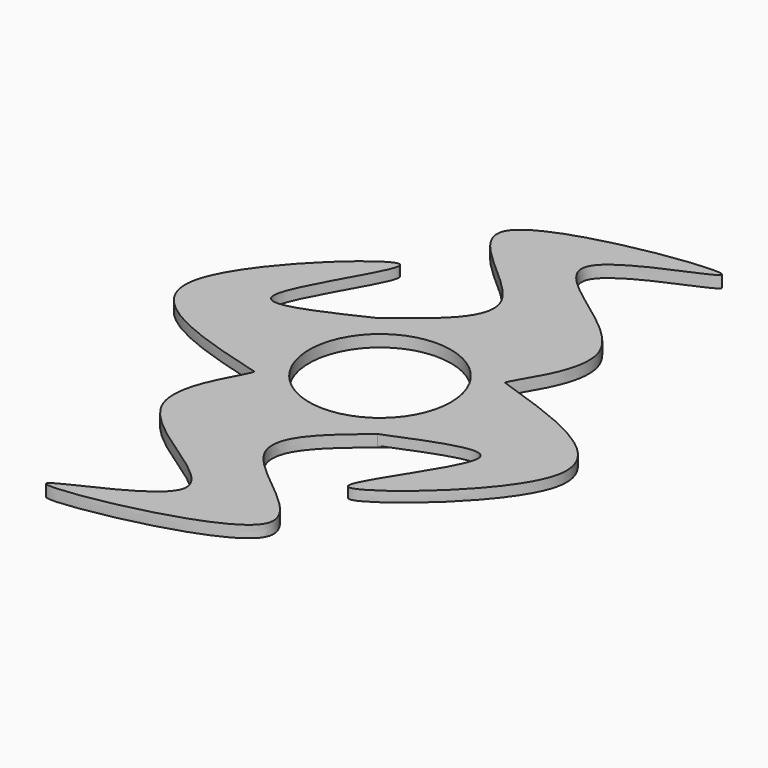
from build123d import *

# Parameters (mm, degrees)
F0_R     = 12.1883906552
F1_DEPTH = 2.032
F3_DEPTH = 1.778
F4_DEPTH = 1.778


with BuildPart() as f1:
    # F0 (on Top) → F1 (new body)
    with BuildSketch(Plane.XY):
        with BuildLine():
            ThreePointArc((13.784794663, 11.0490757015), (18.6441823929, 16.9701638295), (20.38356619, 24.4298875332))
            ThreePointArc((20.38356619, 24.4298875332), (19.8161332392, 28.7679379047), (18.1520153348, 32.8140932132))
            add(Edge.make_bspline(
                [(17.8156372773, 33.3756785813), (17.7587571399, 33.0323279211), (17.952126379, 32.9212248426), (18.1520153348, 32.8140932132)],
                knots=[0.9712656622, 0.9712656622, 0.9712656622, 0.9712656622, 1, 1, 1, 1], degree=3))
            ThreePointArc((17.8156372773, 33.3756785813), (6.8009728243, 40.9732096058), (-6.2803293264, 38.1580995332))
            ThreePointArc((-6.2803293264, 38.1580995332), (-13.0445489471, 27.6172150971), (-10.6757038543, 15.3186995486))
            add(Edge.make_bspline(
                [(-10.4234037199, 14.9371527699), (-10.4293374494, 15.1422077576), (-10.5403253974, 15.2422499293), (-10.6757038543, 15.3186995486)],
                knots=[0.974574343, 0.974574343, 0.974574343, 0.974574343, 0.9946869202, 0.9946869202, 0.9946869202, 0.9946869202], degree=3))
            ThreePointArc((-10.4234037199, 14.9371527699), (0.8429823205, 7.7772901173), (13.784794663, 11.0490757015))
        make_face()
        with Locations((3.5175548401, 24.4298875332)):
            Circle(F0_R, mode=Mode.SUBTRACT)
        with BuildLine():
            add(Edge.make_bspline(
                [(17.8156372773, 33.3756785813), (17.7587571399, 33.0323279211), (17.952126379, 32.9212248426), (18.1520153348, 32.8140932132)],
                knots=[0.9712656622, 0.9712656622, 0.9712656622, 0.9712656622, 1, 1, 1, 1], degree=3))
            ThreePointArc((18.1520153348, 32.8140932132), (17.9865511653, 33.0965180317), (17.8156372773, 33.3756785813))
        make_face()
        with BuildLine():
            add(Edge.make_bspline(
                [(13.784794663, 11.0490757015), (8.3557158887, 6.6054344485), (-3.123614094, -2.9771913197), (36.5265902894, -20.8497673339), (-31.3652954139, -32.9623022839), (18.773370022, -16.8770910693), (-23.9739059772, -3.5018039537), (-10.5024070902, 13.331730969), (-10.4224296856, 14.9034925565), (-10.4234037199, 14.9371527699)],
                knots=[0, 0, 0, 0, 0.1423668823, 0.3032733845, 0.5029627697, 0.6549634449, 0.8323648853, 0.9712728206, 0.974574343, 0.974574343, 0.974574343, 0.974574343], degree=3))
            ThreePointArc((13.784794663, 11.0490757015), (0.8429823205, 7.7772901173), (-10.4234037199, 14.9371527699))
        make_face()
        with BuildLine():
            ThreePointArc((-6.2803293264, 38.1580995332), (6.8009728243, 40.9732096058), (17.8156372773, 33.3756785813))
            add(Edge.make_bspline(
                [(-6.2803293264, 38.1580995332), (-0.6962177807, 42.3878608858), (11.2022462073, 51.4133875551), (-27.7770382027, 70.8090727538), (40.5385488074, 80.3403187132), (-10.1736711582, 66.1577693895), (32.0407127539, 51.1817811584), (18.0906765472, 35.0359227231), (17.8156372773, 33.3756785813)],
                knots=[0, 0, 0, 0, 0.1421531737, 0.3030997713, 0.5028389159, 0.6548774673, 0.8323231132, 0.9712656622, 0.9712656622, 0.9712656622, 0.9712656622], degree=3))
        make_face()
        with BuildLine():
            ThreePointArc((-10.6757038543, 15.3186995486), (-10.5508473299, 15.1270707962), (-10.4234037199, 14.9371527699))
            add(Edge.make_bspline(
                [(-10.4234037199, 14.9371527699), (-10.4293374494, 15.1422077576), (-10.5403253974, 15.2422499293), (-10.6757038543, 15.3186995486)],
                knots=[0.974574343, 0.974574343, 0.974574343, 0.974574343, 0.9946869202, 0.9946869202, 0.9946869202, 0.9946869202], degree=3))
        make_face()
    extrude(amount=F1_DEPTH)

    # F2 (on face) → F3 (join)
    with BuildSketch(Plane.XY.offset(2.032)):
        with BuildLine():
            add(Edge.make_bspline(
                [(-10.4239492892, 14.8876568601), (-22.7152611751, 18.3018164314), (-47.3375447394, 25.2075702094), (-2.6982117701, 64.7380350008), (-30.3618527682, 26.4685111846), (-14.7214727439, 33.8049091648), (-7.3798347824, 37.3026975711)],
                knots=[0.0009667541, 0.0009667541, 0.0009667541, 0.0009667541, 0.2792715137, 0.5603669642, 0.7927469234, 1, 1, 1, 1], degree=3))
            add(Edge.make_bspline(
                [(-10.4234037199, 14.9371527699), (-10.4229448321, 14.9212947447), (-10.4231142501, 14.9048086615), (-10.4239492828, 14.8876568611)],
                knots=[0.9946869202, 0.9946869202, 0.9946869202, 0.9946869202, 0.996242336, 0.996242336, 0.996242336, 0.996242336], degree=3))
            ThreePointArc((-10.4234037199, 14.9371527699), (-13.1944254038, 26.7041028231), (-7.3798347824, 37.3026975711))
        make_face()
    extrude(amount=-F3_DEPTH)

    # F2 (on face) → F4 (join)
    with BuildSketch(Plane.XY.offset(2.032)):
        with BuildLine():
            add(Edge.make_bspline(
                [(17.8156372773, 33.3756785813), (29.9576306347, 29.3100761848), (54.3209173377, 21.1523187318), (7.6315357023, -16.0589632681), (37.2245832749, 20.7510992169), (21.2910187293, 14.1559963145), (13.784794663, 11.0490757015)],
                knots=[0, 0, 0, 0, 0.2793476276, 0.5605196891, 0.7929629822, 1, 1, 1, 1], degree=3))
            ThreePointArc((17.8156372773, 33.3756785813), (20.1152373131, 21.4333436268), (13.784794663, 11.0490757015))
        make_face()
    extrude(amount=-F4_DEPTH)


solid = f1.part
